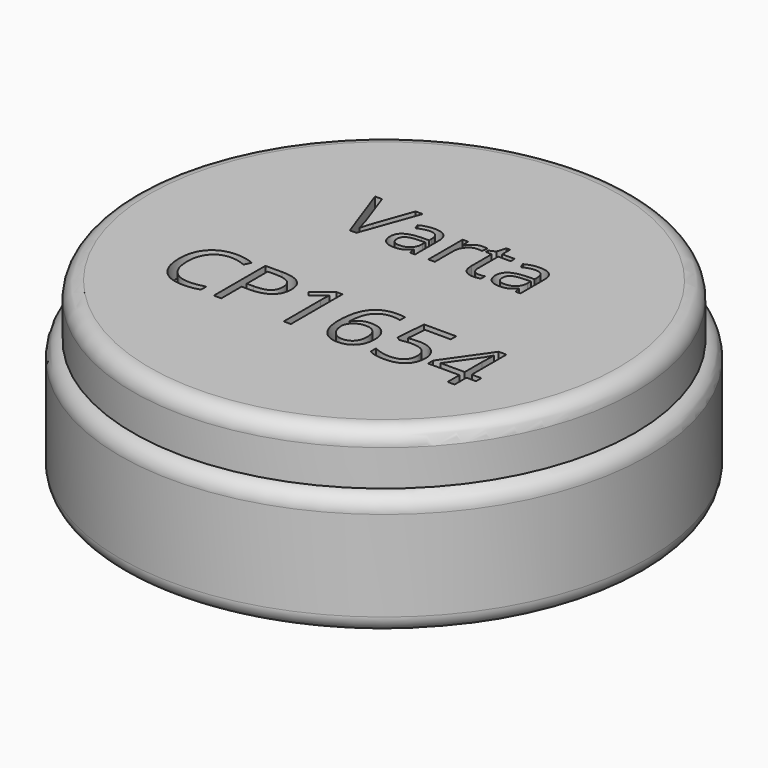
from build123d import *

# Parameters (mm, degrees)
F0_R           = 7.675
F1_DEPTH       = 1.6
F2_TEXT_SIZE   = 2.4466962916
F2_TEXT_SIZE_2 = 2.7623989606
F3_DEPTH       = 0.5
F4_R           = 8.075
F5_DEPTH       = 3.75


# Not quite as in the source:
# - a fillet or chamfer that OpenCascade refuses, or shapes differently, is made with other operations: its cross-section is extruded or revolved along the edge and cut away or added
# - Text() gives the source's letters only with a copy of the font that has no kerning and outlines rounded to 1/6400 em; it was checked with that copy


with BuildPart() as f1:
    # F0 (on Top) → F1 (new body)
    with BuildSketch(Plane.XY):
        Circle(F0_R)
    extrude(amount=F1_DEPTH)

    # F2 (on face) → F3 (cut)
    with BuildSketch(Plane.XY.offset(1.6)):
        with Locations((-2.8883271152, 1.5212824801)):
            Text('Varta', F2_TEXT_SIZE, font='Open Sans', text_align=(TextAlign.LEFT, TextAlign.BOTTOM))
        with Locations((-4.7067750711, -3.1384900212)):
            Text('CP1654', F2_TEXT_SIZE_2, font='Open Sans', text_align=(TextAlign.LEFT, TextAlign.BOTTOM))
    extrude(amount=-F3_DEPTH, mode=Mode.SUBTRACT)

    # F4 (on face) → F5 (join)
    with BuildSketch(Plane(origin=(0, 0, 0), x_dir=(1, 0, 0), z_dir=(0, 0, -1))):
        Circle(F4_R)
    extrude(amount=F5_DEPTH)

    # F6: fillet of radius 0.5 on 3 edges, made by hand

    # F6_s1 → F6_t2 (revolve, cut)
    with BuildSketch(Plane.XZ):
        with BuildLine():
            ThreePointArc((7.675, 1.1), (7.5285533906, 1.4535533906), (7.175, 1.6))
            Line((7.175, 1.6), (7.675, 1.6))
            Line((7.675, 1.6), (7.675, 1.1))
        make_face()
    revolve(axis=Axis((0, 0, 1.6), (0, 0, 1)), mode=Mode.SUBTRACT)

    # F6_s3 → F6_t4 (revolve, cut)
    with BuildSketch(Plane.XZ):
        with BuildLine():
            ThreePointArc((8.075, -0.4898979486), (7.9622983346, -0.1736701825), (7.675, 0))
            Line((7.675, 0), (8.075, 0))
            Line((8.075, 0), (8.075, -0.4898979486))
        make_face()
    revolve(axis=Axis((0, 0, 0), (0, 0, -1)), mode=Mode.SUBTRACT)

    # F6_s5 → F6_t6 (revolve, cut)
    with BuildSketch(Plane.XZ):
        with BuildLine():
            ThreePointArc((8.075, -3.25), (7.9285533906, -3.6035533906), (7.575, -3.75))
            Line((7.575, -3.75), (8.075, -3.75))
            Line((8.075, -3.75), (8.075, -3.25))
        make_face()
    revolve(axis=Axis((0, 0, -3.75), (0, 0, -1)), mode=Mode.SUBTRACT)


solid = f1.part
